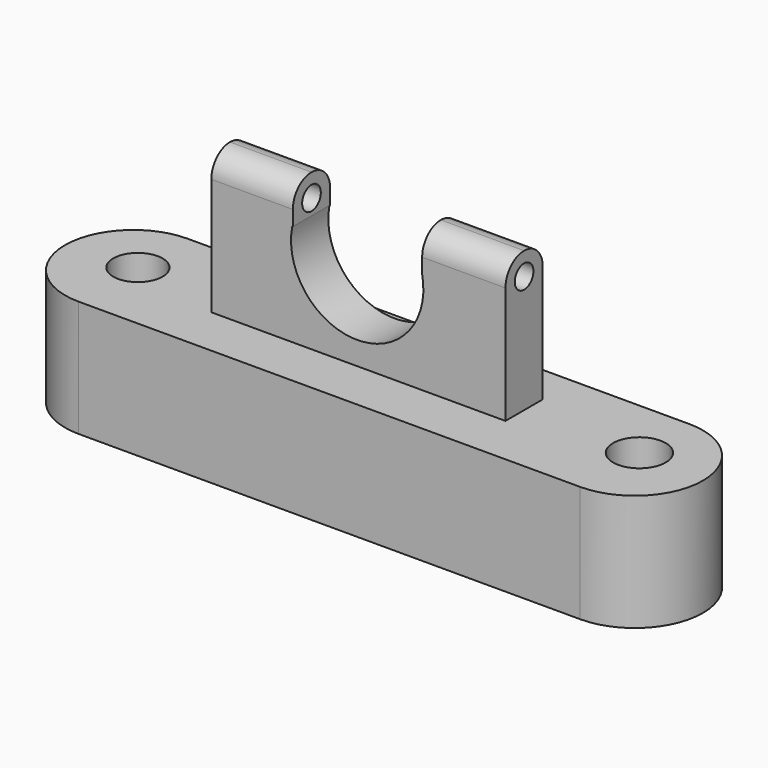
from build123d import *

# Parameters (mm, degrees)
F0_R          = 5.3062476442
F0_R_2        = 5.6471789454
F2_DEPTH      = 25
F3_DEPTH      = 5
F3_DEPTH_BACK = 5
F5_D          = 5
F6_R          = 4.99999


# Not quite as in the source:
# - a fillet or chamfer is up to 0.001 mm smaller than in the source, because OpenCascade refuses the exact size


with BuildPart() as f2:
    # F0 (on Top) → F2 (new body)
    with BuildSketch(Plane.XY):
        with BuildLine():
            Line((55.3750023246, 13.3750010282), (-52.2500015795, 13.3750010282))
            ThreePointArc((-52.2500015795, 13.3750010282), (-66.8750023469, -1.2499997392), (-52.2500015795, -15.8750005066))
            Line((-52.2500015795, -15.8750005066), (55.3750023246, -15.8750005066))
            ThreePointArc((55.3750023246, -15.8750005066), (70.000003092, -1.2499997392), (55.3750023246, 13.3750010282))
        make_face()
        with Locations((-52.2500015795, 0)):
            Circle(F0_R, mode=Mode.SUBTRACT)
        with Locations((55.3750023246, 0)):
            Circle(F0_R_2, mode=Mode.SUBTRACT)
    extrude(amount=-F2_DEPTH)

    # F1 (on Front) → F3 (join, two sides)
    with BuildSketch(Plane.XZ) as f3_sk:
        with BuildLine():
            Line((-32.5000025332, 21.8750014901), (-32.5000025332, 0))
            Line((-32.5000025332, 0), (30.625000596, 0))
            Line((30.625000596, 0), (30.625000596, 21.8750014901))
            Line((30.625000596, 21.8750014901), (30.625000596, 30.1250014454))
            Line((30.625000596, 30.1250014454), (12.7500016242, 30.1250014454))
            Line((12.7500016242, 30.1250014454), (12.7500016242, 21.8750014901))
            ThreePointArc((12.7500016242, 21.8750014901), (-1.1874996126, 4.9502638014), (-15.1250008494, 21.8750014901))
            Line((-15.1250008494, 21.8750014901), (-15.000000596, 21.8750014901))
            Line((-15.000000596, 21.8750014901), (-15.000000596, 30.1250014454))
            Line((-15.000000596, 30.1250014454), (-32.5000025332, 30.1250014454))
            Line((-32.5000025332, 30.1250014454), (-32.5000025332, 21.8750014901))
        make_face()
    extrude(amount=F3_DEPTH)
    extrude(f3_sk.sketch, amount=-F3_DEPTH_BACK)

    # F5 (through all)
    with Locations(Plane(origin=(-32.5000025332, 0, 0), x_dir=(0, -1, 0), z_dir=(-1, 0, 0))):
        with Locations((0, 25.2500027418)):
            Hole(F5_D / 2)

    # F6 (radius 5 in the source; OpenCascade refuses exactly that, so slightly less here)
    f6_edges = [f2.edges().sort_by_distance(p)[0] for p in [
        (21.687501, 5, 30.125001),
        (21.687501, -5, 30.125001),
        (-23.750002, 5, 30.125001),
        (-23.750002, -5, 30.125001),
    ]]
    fillet(f6_edges, radius=F6_R)


solid = f2.part
